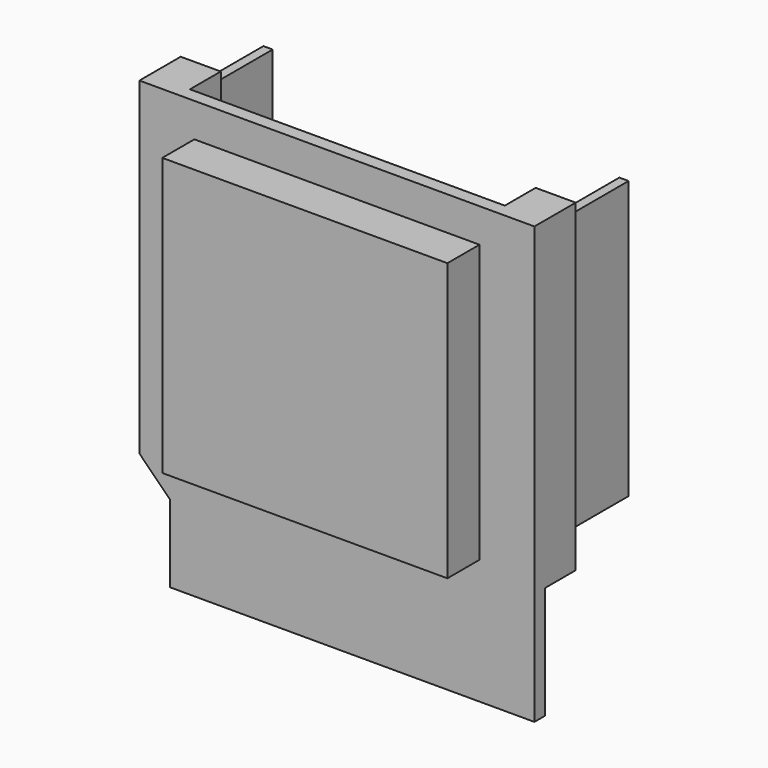
from build123d import *

# Parameters (mm, degrees)
F0_W      = 25.63
F0_H      = 28.3
F1_DEPTH  = 0.85
F2_W      = 9.25
F2_H      = 18
F3_DEPTH  = 2.6
F4_W      = 2
F4_H      = 7
F5_DEPTH  = 25
F6_SIZE   = 1.99999
F7_W      = 2.6
F7_H      = 21
F8_DEPTH  = 2.5
F9_W      = 0.6
F9_H      = 18
F10_DEPTH = 5.5


# Not quite as in the source:
# - a fillet or chamfer is up to 0.001 mm smaller than in the source, because OpenCascade refuses the exact size


with BuildPart() as f1:
    # F0 (on Front) → F1 (new body)
    with BuildSketch(Plane.XZ):
        with Locations((12.815, -14.15)):
            Rectangle(F0_W, F0_H)
    extrude(amount=F1_DEPTH)

    # F2 (on face) → F3 (join)
    with BuildSketch(Plane.XZ.offset(0.85)):
        with Locations((8.19, -11.2)):
            Rectangle(F2_W, F2_H)
        with Locations((17.44, -11.2)):
            Rectangle(F2_W, F2_H)
    extrude(amount=F3_DEPTH)

    # F4 (on face) → F5 (cut)
    with BuildSketch(Plane.XZ.offset(0.85)):
        with Locations((1, -24.8)):
            Rectangle(F4_W, F4_H)
    extrude(amount=-F5_DEPTH, mode=Mode.SUBTRACT)

    # F6 (size 2 in the source; OpenCascade refuses exactly that, so slightly less here)
    f6_edges = [f1.edges().sort_by_distance(p)[0] for p in [
        (2, -0.425, -21.3),
    ]]
    chamfer(f6_edges, length=F6_SIZE)

    # F7 (on face) → F8 (join)
    with BuildSketch(Plane(origin=(0, 0, 0), x_dir=(-1, 0, 0), z_dir=(0, 1, 0))):
        with Locations((-1.3, -10.5)):
            Rectangle(F7_W, F7_H)
        with Locations((-24.33, -10.5)):
            Rectangle(F7_W, F7_H)
    extrude(amount=F8_DEPTH)

    # F9 (on face) → F10 (join)
    with BuildSketch(Plane(origin=(0, 2.5, 0), x_dir=(-1, 0, 0), z_dir=(0, 1, 0))):
        with Locations((-1.2680477372, -10.3143126089)):
            Rectangle(F9_W, F9_H)
        with Locations((-24.3619522628, -10.3143126089)):
            Rectangle(F9_W, F9_H)
    extrude(amount=F10_DEPTH)


solid = f1.part
